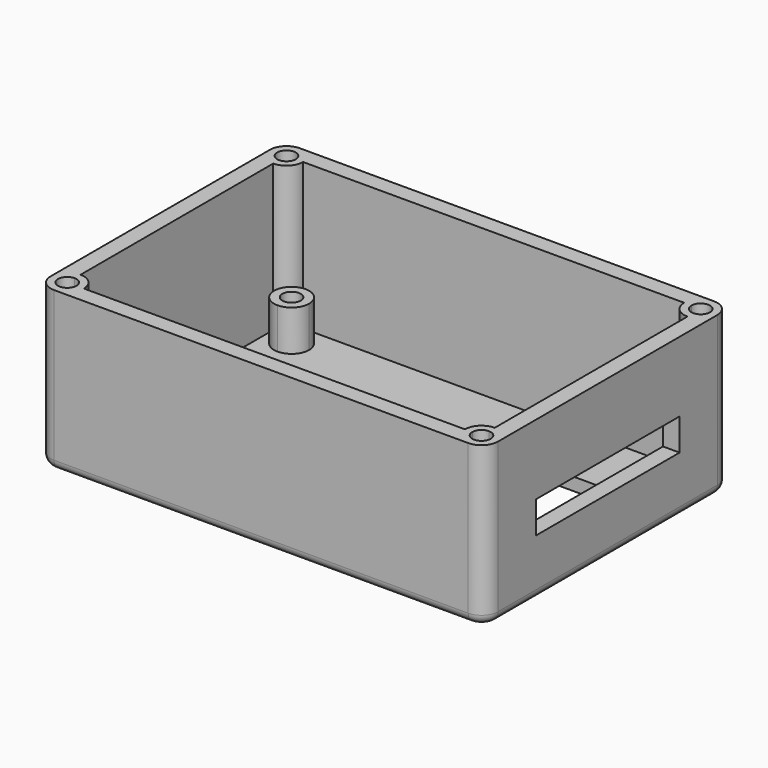
from build123d import *

# Parameters (mm, degrees)
F0_R     = 2.15
F0_W     = 33
F0_H     = 17.6
F1_DEPTH = 2
F2_DEPTH = 25
F3_DEPTH = 8.4
F4_DEPTH = 25
F5_R     = 1.5
F6_W     = 28.2
F6_H     = 5
F7_DEPTH = 3.5


# Not quite as in the source:
# - a feature names something its author has since deleted; it is built from what else it names


with BuildPart() as f1:
    # F0 (on Top) → F1 (new body)
    with BuildSketch(Plane.XY):
        with BuildLine():
            Line((-29.9, -21.5), (29.9, -21.5))
            ThreePointArc((29.9, -21.5), (30.6615223689, -19.6615223689), (32.5, -18.9))
            Line((32.5, -18.9), (32.5, 18.9))
            ThreePointArc((32.5, 18.9), (30.6615223689, 19.6615223689), (29.9, 21.5))
            Line((29.9, 21.5), (-29.9, 21.5))
            ThreePointArc((-29.9, 21.5), (-30.6615223689, 19.6615223689), (-32.5, 18.9))
            Line((-32.5, 18.9), (-32.5, -18.9))
            ThreePointArc((-32.5, -18.9), (-30.6615223689, -19.6615223689), (-29.9, -21.5))
        make_face()
        with BuildLine():
            Line((25.75, -17.5), (-25.75, -17.5))
            ThreePointArc((-25.75, -17.5), (-30.4445436483, -19.4445436483), (-28.5, -14.75))
            Line((-28.5, -14.75), (-28.5, 14.75))
            ThreePointArc((-28.5, 14.75), (-30.4445436483, 19.4445436483), (-25.75, 17.5))
            Line((-25.75, 17.5), (28.5, 17.5))
            Line((28.5, 17.5), (28.5, -14.75))
            ThreePointArc((28.5, -14.75), (30.4445436483, -15.5554563517), (31.25, -17.5))
            ThreePointArc((31.25, -17.5), (28.5, -20.25), (25.75, -17.5))
        make_face(mode=Mode.SUBTRACT)
        with BuildLine():
            ThreePointArc((-28.5, -14.75), (-26.5554563517, -15.5554563517), (-25.75, -17.5))
            Line((-25.75, -17.5), (25.75, -17.5))
            ThreePointArc((25.75, -17.5), (26.5554563517, -15.5554563517), (28.5, -14.75))
            Line((28.5, -14.75), (28.5, 17.5))
            Line((28.5, 17.5), (-25.75, 17.5))
            ThreePointArc((-25.75, 17.5), (-26.5554563517, 15.5554563517), (-28.5, 14.75))
            Line((-28.5, 14.75), (-28.5, -14.75))
        make_face()
        with Locations((-22.5, -12.1)):
            Circle(F0_R, mode=Mode.SUBTRACT)
        with BuildLine():
            ThreePointArc((-16.5527529889, 0.4), (-27.65, 1.9), (-16.5527529889, 3.4))
            Line((-16.5527529889, 3.4), (-14.5, 3.4))
            Line((-14.5, 3.4), (-14.5, 0.4))
            Line((-14.5, 0.4), (-16.5527529889, 0.4))
        make_face(mode=Mode.SUBTRACT)
        with Locations((8, 2.7)):
            Rectangle(F0_W, F0_H, mode=Mode.SUBTRACT)
        with BuildLine():
            Line((-32.4999999696, -24.1), (32.5, -24.1))
            ThreePointArc((32.5, -24.1), (30.6615223689, -23.3384776311), (29.9, -21.5))
            Line((29.9, -21.5), (-29.9, -21.5))
            ThreePointArc((-29.9, -21.5), (-30.6615223582, -23.3384776203), (-32.4999999696, -24.1))
        make_face()
        with BuildLine():
            ThreePointArc((29.9, 21.5), (30.6615223689, 23.3384776311), (32.5, 24.1))
            Line((32.5, 24.1), (-32.5, 24.1))
            ThreePointArc((-32.5, 24.1), (-30.6615223689, 23.3384776311), (-29.9, 21.5))
            Line((-29.9, 21.5), (29.9, 21.5))
        make_face()
        with BuildLine():
            Line((-35.1, 21.5), (-35.1, -21.5))
            ThreePointArc((-35.1, -21.5), (-34.3384776311, -19.6615223689), (-32.5, -18.9))
            Line((-32.5, -18.9), (-32.5, 18.9))
            ThreePointArc((-32.5, 18.9), (-34.3384776311, 19.6615223689), (-35.1, 21.5))
        make_face()
        with BuildLine():
            ThreePointArc((32.5, -18.9), (34.3384776311, -19.6615223689), (35.1, -21.5))
            Line((35.1, -21.5), (35.1, 21.5))
            ThreePointArc((35.1, 21.5), (34.3384776311, 19.6615223689), (32.5, 18.9))
            Line((32.5, 18.9), (32.5, -18.9))
        make_face()
        with BuildLine():
            ThreePointArc((-28.5, -14.75), (-30.4445436483, -19.4445436483), (-25.75, -17.5))
            Line((-25.75, -17.5), (-27.05, -17.5))
            ThreePointArc((-27.05, -17.5), (-29.5253048327, -18.5253048327), (-28.5, -16.05))
            Line((-28.5, -16.05), (-28.5, -14.75))
        make_face()
        with BuildLine():
            ThreePointArc((-25.75, 17.5), (-30.4445436483, 19.4445436483), (-28.5, 14.75))
            Line((-28.5, 14.75), (-28.5, 16.05))
            ThreePointArc((-28.5, 16.05), (-29.5253048327, 18.5253048327), (-27.05, 17.5))
            Line((-27.05, 17.5), (-25.75, 17.5))
        make_face()
        with BuildLine():
            Line((27.05, -17.5), (25.75, -17.5))
            ThreePointArc((25.75, -17.5), (28.5, -20.25), (31.25, -17.5))
            ThreePointArc((31.25, -17.5), (30.4445436483, -15.5554563517), (28.5, -14.75))
            Line((28.5, -14.75), (28.5, -16.05))
            ThreePointArc((28.5, -16.05), (29.5253048327, -16.4746951673), (29.95, -17.5))
            ThreePointArc((29.95, -17.5), (28.5, -18.95), (27.05, -17.5))
        make_face()
        with BuildLine():
            ThreePointArc((-35.1, -21.5), (-34.3384776203, -23.3384776418), (-32.4999999696, -24.1))
            ThreePointArc((-32.4999999696, -24.1), (-30.6615223582, -23.3384776203), (-29.9, -21.5))
            Line((-29.9, -21.5), (-31.05, -21.5))
            ThreePointArc((-31.05, -21.5), (-33.5253048327, -22.5253048327), (-32.5, -20.05))
            Line((-32.5, -20.05), (-32.5, -18.9))
            ThreePointArc((-32.5, -18.9), (-34.3384776311, -19.6615223689), (-35.1, -21.5))
        make_face()
        with BuildLine():
            ThreePointArc((32.5, 18.9), (34.3384776311, 19.6615223689), (35.1, 21.5))
            ThreePointArc((35.1, 21.5), (34.3384776311, 23.3384776311), (32.5, 24.1))
            ThreePointArc((32.5, 24.1), (30.6615223689, 23.3384776311), (29.9, 21.5))
            Line((29.9, 21.5), (31.05, 21.5))
            ThreePointArc((31.05, 21.5), (32.5, 22.95), (33.95, 21.5))
            ThreePointArc((33.95, 21.5), (33.5253048327, 20.4746951673), (32.5, 20.05))
            Line((32.5, 20.05), (32.5, 18.9))
        make_face()
        with BuildLine():
            ThreePointArc((-32.5, 24.1), (-34.3384776311, 23.3384776311), (-35.1, 21.5))
            ThreePointArc((-35.1, 21.5), (-34.3384776311, 19.6615223689), (-32.5, 18.9))
            Line((-32.5, 18.9), (-32.5, 20.05))
            ThreePointArc((-32.5, 20.05), (-33.5253048327, 22.5253048327), (-31.05, 21.5))
            Line((-31.05, 21.5), (-29.9, 21.5))
            ThreePointArc((-29.9, 21.5), (-30.6615223689, 23.3384776311), (-32.5, 24.1))
        make_face()
        with BuildLine():
            ThreePointArc((29.9, -21.5), (30.6615223689, -23.3384776311), (32.5, -24.1))
            ThreePointArc((32.5, -24.1), (34.3384776311, -23.3384776311), (35.1, -21.5))
            ThreePointArc((35.1, -21.5), (34.3384776311, -19.6615223689), (32.5, -18.9))
            Line((32.5, -18.9), (32.5, -20.05))
            ThreePointArc((32.5, -20.05), (33.5253048327, -20.4746951673), (33.95, -21.5))
            ThreePointArc((33.95, -21.5), (32.5, -22.95), (31.05, -21.5))
            Line((31.05, -21.5), (29.9, -21.5))
        make_face()
        with BuildLine():
            ThreePointArc((-28.5, -16.05), (-29.5253048327, -18.5253048327), (-27.05, -17.5))
            Line((-27.05, -17.5), (-28.5, -17.5))
            Line((-28.5, -17.5), (-28.5, -16.05))
        make_face()
        with BuildLine():
            ThreePointArc((-32.5, -20.05), (-33.5253048327, -22.5253048327), (-31.05, -21.5))
            Line((-31.05, -21.5), (-32.5, -21.5))
            Line((-32.5, -21.5), (-32.5, -20.05))
        make_face()
        with BuildLine():
            Line((32.5, 21.5), (32.5, 20.05))
            ThreePointArc((32.5, 20.05), (33.5253048327, 20.4746951673), (33.95, 21.5))
            ThreePointArc((33.95, 21.5), (32.5, 22.95), (31.05, 21.5))
            Line((31.05, 21.5), (32.5, 21.5))
        make_face()
        with BuildLine():
            ThreePointArc((-31.05, 21.5), (-33.5253048327, 22.5253048327), (-32.5, 20.05))
            Line((-32.5, 20.05), (-32.5, 21.5))
            Line((-32.5, 21.5), (-31.05, 21.5))
        make_face()
        with BuildLine():
            Line((32.5, -21.5), (31.05, -21.5))
            ThreePointArc((31.05, -21.5), (32.5, -22.95), (33.95, -21.5))
            ThreePointArc((33.95, -21.5), (33.5253048327, -20.4746951673), (32.5, -20.05))
            Line((32.5, -20.05), (32.5, -21.5))
        make_face()
        with BuildLine():
            ThreePointArc((-27.05, 17.5), (-29.5253048327, 18.5253048327), (-28.5, 16.05))
            Line((-28.5, 16.05), (-28.5, 17.5))
            Line((-28.5, 17.5), (-27.05, 17.5))
        make_face()
        with BuildLine():
            Line((28.5, -17.5), (27.05, -17.5))
            ThreePointArc((27.05, -17.5), (28.5, -18.95), (29.95, -17.5))
            ThreePointArc((29.95, -17.5), (29.5253048327, -16.4746951673), (28.5, -16.05))
            Line((28.5, -16.05), (28.5, -17.5))
        make_face()
        with BuildLine():
            Line((-27.05, -17.5), (-25.75, -17.5))
            ThreePointArc((-25.75, -17.5), (-26.5554563517, -15.5554563517), (-28.5, -14.75))
            Line((-28.5, -14.75), (-28.5, -16.05))
            ThreePointArc((-28.5, -16.05), (-27.4746951673, -16.4746951673), (-27.05, -17.5))
        make_face()
        with BuildLine():
            Line((-28.5, 16.05), (-28.5, 14.75))
            ThreePointArc((-28.5, 14.75), (-26.5554563517, 15.5554563517), (-25.75, 17.5))
            Line((-25.75, 17.5), (-27.05, 17.5))
            ThreePointArc((-27.05, 17.5), (-27.4746951673, 16.4746951673), (-28.5, 16.05))
        make_face()
        with BuildLine():
            ThreePointArc((28.5, -14.75), (26.5554563517, -15.5554563517), (25.75, -17.5))
            Line((25.75, -17.5), (27.05, -17.5))
            ThreePointArc((27.05, -17.5), (27.4746951673, -16.4746951673), (28.5, -16.05))
            Line((28.5, -16.05), (28.5, -14.75))
        make_face()
        with BuildLine():
            Line((-31.05, -21.5), (-29.9, -21.5))
            ThreePointArc((-29.9, -21.5), (-30.6615223689, -19.6615223689), (-32.5, -18.9))
            Line((-32.5, -18.9), (-32.5, -20.05))
            ThreePointArc((-32.5, -20.05), (-31.4746951673, -20.4746951673), (-31.05, -21.5))
        make_face()
        with BuildLine():
            ThreePointArc((29.9, 21.5), (30.6615223689, 19.6615223689), (32.5, 18.9))
            Line((32.5, 18.9), (32.5, 20.05))
            ThreePointArc((32.5, 20.05), (31.4746951673, 20.4746951673), (31.05, 21.5))
            Line((31.05, 21.5), (29.9, 21.5))
        make_face()
        with BuildLine():
            Line((-32.5, 20.05), (-32.5, 18.9))
            ThreePointArc((-32.5, 18.9), (-30.6615223689, 19.6615223689), (-29.9, 21.5))
            Line((-29.9, 21.5), (-31.05, 21.5))
            ThreePointArc((-31.05, 21.5), (-31.4746951673, 20.4746951673), (-32.5, 20.05))
        make_face()
        with BuildLine():
            ThreePointArc((32.5, -18.9), (30.6615223689, -19.6615223689), (29.9, -21.5))
            Line((29.9, -21.5), (31.05, -21.5))
            ThreePointArc((31.05, -21.5), (31.4746951673, -20.4746951673), (32.5, -20.05))
            Line((32.5, -20.05), (32.5, -18.9))
        make_face()
        with BuildLine():
            Line((-28.5, -17.5), (-27.05, -17.5))
            ThreePointArc((-27.05, -17.5), (-27.4746951673, -16.4746951673), (-28.5, -16.05))
            Line((-28.5, -16.05), (-28.5, -17.5))
        make_face()
        with BuildLine():
            Line((-32.5, -21.5), (-31.05, -21.5))
            ThreePointArc((-31.05, -21.5), (-31.4746951673, -20.4746951673), (-32.5, -20.05))
            Line((-32.5, -20.05), (-32.5, -21.5))
        make_face()
        with BuildLine():
            ThreePointArc((31.05, 21.5), (31.4746951673, 20.4746951673), (32.5, 20.05))
            Line((32.5, 20.05), (32.5, 21.5))
            Line((32.5, 21.5), (31.05, 21.5))
        make_face()
        with BuildLine():
            Line((-32.5, 21.5), (-32.5, 20.05))
            ThreePointArc((-32.5, 20.05), (-31.4746951673, 20.4746951673), (-31.05, 21.5))
            Line((-31.05, 21.5), (-32.5, 21.5))
        make_face()
        with BuildLine():
            ThreePointArc((32.5, -20.05), (31.4746951673, -20.4746951673), (31.05, -21.5))
            Line((31.05, -21.5), (32.5, -21.5))
            Line((32.5, -21.5), (32.5, -20.05))
        make_face()
        with BuildLine():
            Line((-28.5, 17.5), (-28.5, 16.05))
            ThreePointArc((-28.5, 16.05), (-27.4746951673, 16.4746951673), (-27.05, 17.5))
            Line((-27.05, 17.5), (-28.5, 17.5))
        make_face()
        with BuildLine():
            ThreePointArc((28.5, -16.05), (27.4746951673, -16.4746951673), (27.05, -17.5))
            Line((27.05, -17.5), (28.5, -17.5))
            Line((28.5, -17.5), (28.5, -16.05))
        make_face()
    extrude(amount=F1_DEPTH)

    # F0 (on Top) → F2 (join)
    with BuildSketch(Plane.XY):
        with BuildLine():
            Line((-32.5, 20.05), (-32.5, 18.9))
            ThreePointArc((-32.5, 18.9), (-30.6615223689, 19.6615223689), (-29.9, 21.5))
            Line((-29.9, 21.5), (-31.05, 21.5))
            ThreePointArc((-31.05, 21.5), (-31.4746951673, 20.4746951673), (-32.5, 20.05))
        make_face()
        with BuildLine():
            ThreePointArc((-32.5, 24.1), (-34.3384776311, 23.3384776311), (-35.1, 21.5))
            ThreePointArc((-35.1, 21.5), (-34.3384776311, 19.6615223689), (-32.5, 18.9))
            Line((-32.5, 18.9), (-32.5, 20.05))
            ThreePointArc((-32.5, 20.05), (-33.5253048327, 22.5253048327), (-31.05, 21.5))
            Line((-31.05, 21.5), (-29.9, 21.5))
            ThreePointArc((-29.9, 21.5), (-30.6615223689, 23.3384776311), (-32.5, 24.1))
        make_face()
        with BuildLine():
            Line((-35.1, 21.5), (-35.1, -21.5))
            ThreePointArc((-35.1, -21.5), (-34.3384776311, -19.6615223689), (-32.5, -18.9))
            Line((-32.5, -18.9), (-32.5, 18.9))
            ThreePointArc((-32.5, 18.9), (-34.3384776311, 19.6615223689), (-35.1, 21.5))
        make_face()
        with BuildLine():
            ThreePointArc((29.9, 21.5), (30.6615223689, 23.3384776311), (32.5, 24.1))
            Line((32.5, 24.1), (-32.5, 24.1))
            ThreePointArc((-32.5, 24.1), (-30.6615223689, 23.3384776311), (-29.9, 21.5))
            Line((-29.9, 21.5), (29.9, 21.5))
        make_face()
        with BuildLine():
            ThreePointArc((29.9, 21.5), (30.6615223689, 19.6615223689), (32.5, 18.9))
            Line((32.5, 18.9), (32.5, 20.05))
            ThreePointArc((32.5, 20.05), (31.4746951673, 20.4746951673), (31.05, 21.5))
            Line((31.05, 21.5), (29.9, 21.5))
        make_face()
        with BuildLine():
            ThreePointArc((32.5, 18.9), (34.3384776311, 19.6615223689), (35.1, 21.5))
            ThreePointArc((35.1, 21.5), (34.3384776311, 23.3384776311), (32.5, 24.1))
            ThreePointArc((32.5, 24.1), (30.6615223689, 23.3384776311), (29.9, 21.5))
            Line((29.9, 21.5), (31.05, 21.5))
            ThreePointArc((31.05, 21.5), (32.5, 22.95), (33.95, 21.5))
            ThreePointArc((33.95, 21.5), (33.5253048327, 20.4746951673), (32.5, 20.05))
            Line((32.5, 20.05), (32.5, 18.9))
        make_face()
        with BuildLine():
            ThreePointArc((32.5, -18.9), (34.3384776311, -19.6615223689), (35.1, -21.5))
            Line((35.1, -21.5), (35.1, 21.5))
            ThreePointArc((35.1, 21.5), (34.3384776311, 19.6615223689), (32.5, 18.9))
            Line((32.5, 18.9), (32.5, -18.9))
        make_face()
        with BuildLine():
            ThreePointArc((29.9, -21.5), (30.6615223689, -23.3384776311), (32.5, -24.1))
            ThreePointArc((32.5, -24.1), (34.3384776311, -23.3384776311), (35.1, -21.5))
            ThreePointArc((35.1, -21.5), (34.3384776311, -19.6615223689), (32.5, -18.9))
            Line((32.5, -18.9), (32.5, -20.05))
            ThreePointArc((32.5, -20.05), (33.5253048327, -20.4746951673), (33.95, -21.5))
            ThreePointArc((33.95, -21.5), (32.5, -22.95), (31.05, -21.5))
            Line((31.05, -21.5), (29.9, -21.5))
        make_face()
        with BuildLine():
            ThreePointArc((32.5, -18.9), (30.6615223689, -19.6615223689), (29.9, -21.5))
            Line((29.9, -21.5), (31.05, -21.5))
            ThreePointArc((31.05, -21.5), (31.4746951673, -20.4746951673), (32.5, -20.05))
            Line((32.5, -20.05), (32.5, -18.9))
        make_face()
        with BuildLine():
            Line((-32.4999999696, -24.1), (32.5, -24.1))
            ThreePointArc((32.5, -24.1), (30.6615223689, -23.3384776311), (29.9, -21.5))
            Line((29.9, -21.5), (-29.9, -21.5))
            ThreePointArc((-29.9, -21.5), (-30.6615223582, -23.3384776203), (-32.4999999696, -24.1))
        make_face()
        with BuildLine():
            Line((-31.05, -21.5), (-29.9, -21.5))
            ThreePointArc((-29.9, -21.5), (-30.6615223689, -19.6615223689), (-32.5, -18.9))
            Line((-32.5, -18.9), (-32.5, -20.05))
            ThreePointArc((-32.5, -20.05), (-31.4746951673, -20.4746951673), (-31.05, -21.5))
        make_face()
        with BuildLine():
            ThreePointArc((-35.1, -21.5), (-34.3384776203, -23.3384776418), (-32.4999999696, -24.1))
            ThreePointArc((-32.4999999696, -24.1), (-30.6615223582, -23.3384776203), (-29.9, -21.5))
            Line((-29.9, -21.5), (-31.05, -21.5))
            ThreePointArc((-31.05, -21.5), (-33.5253048327, -22.5253048327), (-32.5, -20.05))
            Line((-32.5, -20.05), (-32.5, -18.9))
            ThreePointArc((-32.5, -18.9), (-34.3384776311, -19.6615223689), (-35.1, -21.5))
        make_face()
    extrude(amount=F2_DEPTH)

    # F0 (on Top) → F3 (join)
    with BuildSketch(Plane.XY):
        with BuildLine():
            ThreePointArc((-25.75, 17.5), (-30.4445436483, 19.4445436483), (-28.5, 14.75))
            Line((-28.5, 14.75), (-28.5, 16.05))
            ThreePointArc((-28.5, 16.05), (-29.5253048327, 18.5253048327), (-27.05, 17.5))
            Line((-27.05, 17.5), (-25.75, 17.5))
        make_face()
        with BuildLine():
            Line((-28.5, 16.05), (-28.5, 14.75))
            ThreePointArc((-28.5, 14.75), (-26.5554563517, 15.5554563517), (-25.75, 17.5))
            Line((-25.75, 17.5), (-27.05, 17.5))
            ThreePointArc((-27.05, 17.5), (-27.4746951673, 16.4746951673), (-28.5, 16.05))
        make_face()
        with BuildLine():
            ThreePointArc((28.5, -14.75), (26.5554563517, -15.5554563517), (25.75, -17.5))
            Line((25.75, -17.5), (27.05, -17.5))
            ThreePointArc((27.05, -17.5), (27.4746951673, -16.4746951673), (28.5, -16.05))
            Line((28.5, -16.05), (28.5, -14.75))
        make_face()
        with BuildLine():
            Line((27.05, -17.5), (25.75, -17.5))
            ThreePointArc((25.75, -17.5), (28.5, -20.25), (31.25, -17.5))
            ThreePointArc((31.25, -17.5), (30.4445436483, -15.5554563517), (28.5, -14.75))
            Line((28.5, -14.75), (28.5, -16.05))
            ThreePointArc((28.5, -16.05), (29.5253048327, -16.4746951673), (29.95, -17.5))
            ThreePointArc((29.95, -17.5), (28.5, -18.95), (27.05, -17.5))
        make_face()
        with BuildLine():
            Line((-27.05, -17.5), (-25.75, -17.5))
            ThreePointArc((-25.75, -17.5), (-26.5554563517, -15.5554563517), (-28.5, -14.75))
            Line((-28.5, -14.75), (-28.5, -16.05))
            ThreePointArc((-28.5, -16.05), (-27.4746951673, -16.4746951673), (-27.05, -17.5))
        make_face()
        with BuildLine():
            ThreePointArc((-28.5, -14.75), (-30.4445436483, -19.4445436483), (-25.75, -17.5))
            Line((-25.75, -17.5), (-27.05, -17.5))
            ThreePointArc((-27.05, -17.5), (-29.5253048327, -18.5253048327), (-28.5, -16.05))
            Line((-28.5, -16.05), (-28.5, -14.75))
        make_face()
    extrude(amount=F3_DEPTH)

    # F0 (on Top) → F4 (cut)
    with BuildSketch(Plane.XY):
        with Locations((8, 2.7)):
            Rectangle(F0_W, F0_H)
        with BuildLine():
            Line((-22, 3.4), (-16.5527529889, 3.4))
            ThreePointArc((-16.5527529889, 3.4), (-27.65, 1.9), (-16.5527529889, 0.4))
            Line((-16.5527529889, 0.4), (-22, 0.4))
            Line((-22, 0.4), (-22, 3.4))
        make_face()
        with BuildLine():
            ThreePointArc((-16.5527529889, 0.4), (-16.4009176818, 1.1431795499), (-16.35, 1.9))
            ThreePointArc((-16.35, 1.9), (-16.4009176818, 2.6568204501), (-16.5527529889, 3.4))
            Line((-16.5527529889, 3.4), (-22, 3.4))
            Line((-22, 3.4), (-22, 0.4))
            Line((-22, 0.4), (-16.5527529889, 0.4))
        make_face()
        with Locations((-22.5, -12.1)):
            Circle(F0_R)
    extrude(amount=-F4_DEPTH, mode=Mode.SUBTRACT)

    # F5
    f5_edges = [f1.edges().sort_by_distance(p)[0] for p in [
        (0, 24.1, 0),
    ]]
    fillet(f5_edges, radius=F5_R)

    # F6 (on face) → F7 (cut)
    with BuildSketch(Plane.YZ.offset(35.1)):
        with Locations((0, 11.5)):
            Rectangle(F6_W, F6_H)
    extrude(amount=-F7_DEPTH, mode=Mode.SUBTRACT)


solid = f1.part
